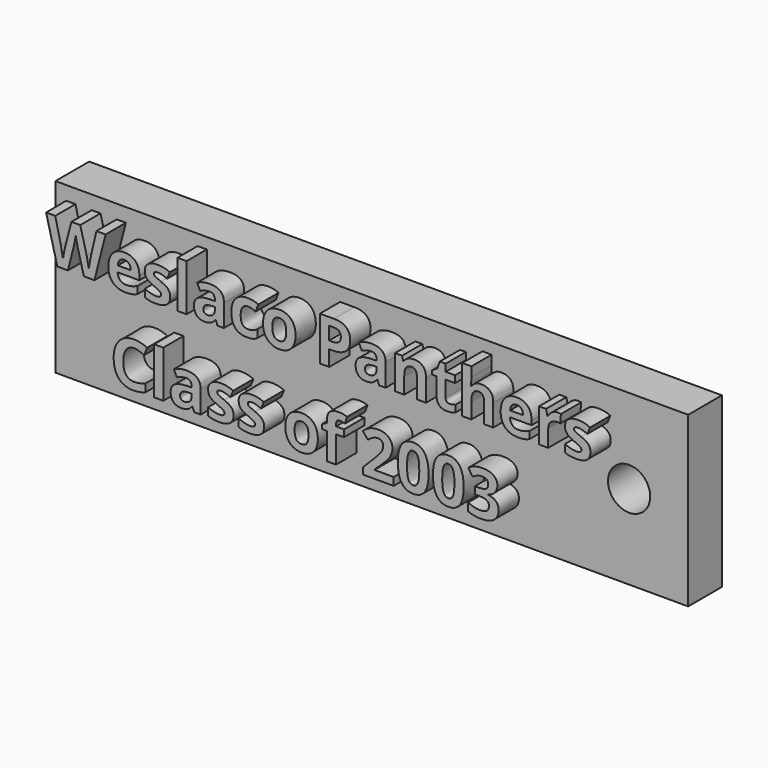
from build123d import *

# Parameters (mm, degrees)
F0_W         = 75
F0_H         = 20
F0_R         = 2.5
F1_DEPTH     = 5
F2_TEXT_SIZE = 7.2981175769
F3_DEPTH     = 3


# Not quite as in the source:
# - Text() gives the source's letters only with a copy of the font that has no kerning and outlines rounded to 1/6400 em; it was checked with that copy


with BuildPart() as f1:
    # F0 (on Front) → F1 (new body)
    with BuildSketch(Plane.XZ):
        with Locations((37.5, -10)):
            Rectangle(F0_W, F0_H)
        with Locations((68, -10)):
            Circle(F0_R, mode=Mode.SUBTRACT)
    extrude(amount=F1_DEPTH)

    # F2 (on face) → F3 (join)
    with BuildSketch(Plane.XZ.offset(5)):
        with Locations((1.2921256625, -6.8482664119)):
            Text('Weslaco Panthers', F2_TEXT_SIZE, font='Open Sans', font_style=FontStyle.BOLD, text_align=(TextAlign.LEFT, TextAlign.BOTTOM))
        with Locations((8.877606619, -16.7737063165)):
            Text('Class of 2003', F2_TEXT_SIZE, font='Open Sans', font_style=FontStyle.BOLD, text_align=(TextAlign.LEFT, TextAlign.BOTTOM))
    extrude(amount=F3_DEPTH)


solid = f1.part
